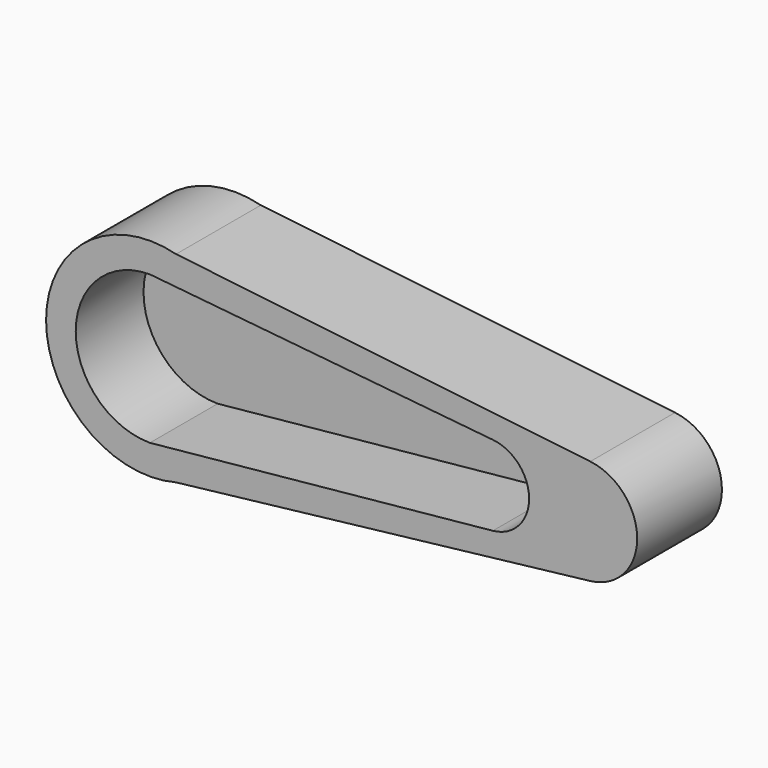
from build123d import *

# Parameters (mm, degrees)
F1_DEPTH = 5
F2_DEPTH = 1


# Not quite as in the source:
# - a feature names something its author has since deleted; it is built from what else it names


with BuildPart() as f1:
    # F0 (on Front) → F1 (new body)
    with BuildSketch(Plane.XZ):
        with BuildLine():
            Line((1.2337693236, -4.7421317207), (20.7868759001, -2.4834859005))
            ThreePointArc((20.7868759001, -2.4834859005), (23, 0), (20.7868759001, 2.4834859005))
            Line((20.7868759001, 2.4834859005), (1.2337693236, 4.7421317207))
            ThreePointArc((1.2337693236, 4.7421317207), (-4.9, 0), (1.2337693236, -4.7421317207))
        make_face()
        with BuildLine():
            ThreePointArc((0, -3.5), (-3.5, 0), (0, 3.5))
            Line((0, 3.5), (16.1879612334, 1.8906799239))
            ThreePointArc((16.1879612334, 1.8906799239), (17.9, 0), (16.1879612334, -1.8906799239))
            Line((16.1879612334, -1.8906799239), (0, -3.5))
        make_face(mode=Mode.SUBTRACT)
    extrude(amount=F1_DEPTH)

    # F0 (on Front) → F2 (join)
    with BuildSketch(Plane.XZ):
        with BuildLine():
            Line((1.2337693236, -4.7421317207), (20.7868759001, -2.4834859005))
            ThreePointArc((20.7868759001, -2.4834859005), (23, 0), (20.7868759001, 2.4834859005))
            Line((20.7868759001, 2.4834859005), (1.2337693236, 4.7421317207))
            ThreePointArc((1.2337693236, 4.7421317207), (-4.9, 0), (1.2337693236, -4.7421317207))
        make_face()
        with BuildLine():
            ThreePointArc((0, -3.5), (-3.5, 0), (0, 3.5))
            Line((0, 3.5), (16.1879612334, 1.8906799239))
            ThreePointArc((16.1879612334, 1.8906799239), (17.9, 0), (16.1879612334, -1.8906799239))
            Line((16.1879612334, -1.8906799239), (0, -3.5))
        make_face(mode=Mode.SUBTRACT)
        with BuildLine():
            Line((16.1879612334, 1.8906799239), (0, 3.5))
            ThreePointArc((0, 3.5), (-3.5, 0), (0, -3.5))
            Line((0, -3.5), (16.1879612334, -1.8906799239))
            ThreePointArc((16.1879612334, -1.8906799239), (17.9, 0), (16.1879612334, 1.8906799239))
        make_face()
    extrude(amount=F2_DEPTH)


solid = f1.part
